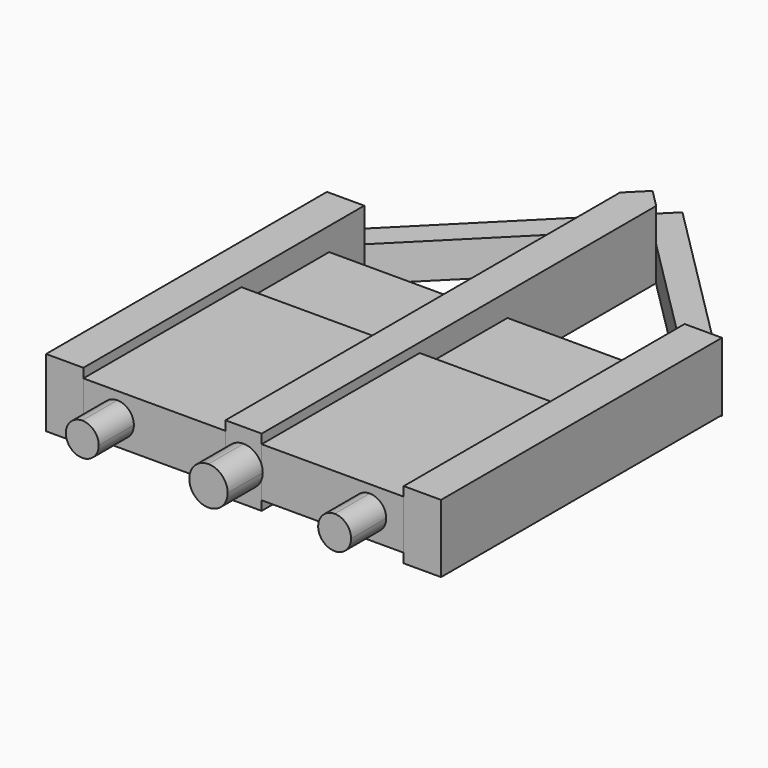
from build123d import *

# Parameters (mm, degrees)
F0_W     = 1.7
F0_H     = 9
F0_H_2   = 2
F0_H_3   = 5
F1_DEPTH = 1.55
F0_W_2   = 0.825
F2_DEPTH = 1.125
F3_DEPTH = 1.6
F0_W_3   = 6.475
F4_DEPTH = 0.5
F0_W_4   = 1.5
F5_DEPTH = 0.75
F6_DEPTH = 0.875
F7_R     = 0.87499
F8_R     = 0.74999
F8_2_R   = 0.74999


# Not quite as in the source:
# - a fillet or chamfer is up to 0.001 mm smaller than in the source, because OpenCascade refuses the exact size


with BuildPart() as f1:
    # F0 (on Top) → F1 (new body, symmetric)
    with BuildSketch(Plane.XY):
        with Locations((0.85, 4.5)):
            Rectangle(F0_W, F0_H)
        with Locations((0.85, 15)):
            Rectangle(F0_W, F0_H_2)
        with Locations((0.85, 11.5)):
            Rectangle(F0_W, F0_H_3)
    extrude(amount=F1_DEPTH, both=True)


with BuildPart() as f1b:
    # F0 (on Top) → F1, piece 2 (new body, symmetric)
    with BuildSketch(Plane.XY):
        with Locations((17.15, 4.5)):
            Rectangle(F0_W, F0_H)
        with Locations((17.15, 15)):
            Rectangle(F0_W, F0_H_2)
        with Locations((17.15, 11.5)):
            Rectangle(F0_W, F0_H_3)
    extrude(amount=F1_DEPTH, both=True)


with BuildPart() as f1c:
    # F0 (on Top) → F1, piece 3 (new body, symmetric)
    with BuildSketch(Plane.XY):
        with Locations((8.5875, 4.5)):
            Rectangle(F0_W_2, F0_H)
        with Locations((9.4125, 4.5)):
            Rectangle(F0_W_2, F0_H)
        with Locations((9.4125, 11.5)):
            Rectangle(F0_W_2, F0_H_3)
        with Locations((8.5875, 11.5)):
            Rectangle(F0_W_2, F0_H_3)
        Polygon((8.175, 22.475), (8.175, 14), (9, 14), (9, 23.3), align=None)
        Polygon((9, 23.3), (9, 14), (9.825, 14), (9.825, 22.475), align=None)
    extrude(amount=F1_DEPTH, both=True)


with BuildPart() as f2:
    # F0 (on Top) → F2 (new body, symmetric)
    with BuildSketch(Plane.XY):
        Polygon((1.7, 9), (1.7, 0), (2.5, 0), (4, 0), (8.125, 0), (8.175, 0), (8.175, 9), align=None)
    extrude(amount=F2_DEPTH, both=True)


with BuildPart() as f2b:
    # F0 (on Top) → F2, piece 2 (new body, symmetric)
    with BuildSketch(Plane.XY):
        Polygon((16.3, 9), (9.825, 9), (9.825, 0), (9.875, 0), (14, 0), (15.5, 0), (16.3, 0), align=None)
    extrude(amount=F2_DEPTH, both=True)


with BuildPart() as f3:
    # F0 (on Top) → F3 (new body)
    with BuildSketch(Plane.XY):
        Polygon((9, 25), (0, 16), (1.7, 16), (8.175, 22.475), (9, 23.3), align=None)
        Polygon((18, 16), (9, 25), (9, 23.3), (9.825, 22.475), (16.3, 16), align=None)
    extrude(amount=-F3_DEPTH)


with BuildPart() as f4:
    # F0 (on Top) → F4 (new body, symmetric)
    with BuildSketch(Plane.XY):
        with Locations((4.9375, 11.5)):
            Rectangle(F0_W_3, F0_H_3)
    extrude(amount=F4_DEPTH, both=True)


with BuildPart() as f4b:
    # F0 (on Top) → F4, piece 2 (new body, symmetric)
    with BuildSketch(Plane.XY):
        with Locations((13.0625, 11.5)):
            Rectangle(F0_W_3, F0_H_3)
    extrude(amount=F4_DEPTH, both=True)


with BuildPart() as f5:
    # F0 (on Top) → F5 (new body, symmetric)
    with BuildSketch(Plane.XY):
        with Locations((3.25, -1)):
            Rectangle(F0_W_4, F0_H_2)
    extrude(amount=F5_DEPTH, both=True)

    # F8#2 (radius 0.75 in the source; OpenCascade refuses exactly that, so slightly less here)
    f8_2_edges = [f5.edges().sort_by_distance(p)[0] for p in [
        (2.5, -1, 0.75),
        (4, -1, 0.75),
        (2.5, -1, -0.75),
        (4, -1, -0.75),
    ]]
    fillet(f8_2_edges, radius=F8_2_R)


with BuildPart() as f5b:
    # F0 (on Top) → F5, piece 2 (new body, symmetric)
    with BuildSketch(Plane.XY):
        with Locations((14.75, -1)):
            Rectangle(F0_W_4, F0_H_2)
    extrude(amount=F5_DEPTH, both=True)

    # F8 (radius 0.75 in the source; OpenCascade refuses exactly that, so slightly less here)
    f8_edges = [f5b.edges().sort_by_distance(p)[0] for p in [
        (14, -1, 0.75),
        (15.5, -1, 0.75),
        (15.5, -1, -0.75),
        (14, -1, -0.75),
    ]]
    fillet(f8_edges, radius=F8_R)


with BuildPart() as f6:
    # F0 (on Top) → F6 (new body, symmetric)
    with BuildSketch(Plane.XY):
        Polygon((8.175, 0), (8.125, 0), (8.125, -2), (9.875, -2), (9.875, 0), (9.825, 0), (9, 0), align=None)
    extrude(amount=F6_DEPTH, both=True)

    # F7 (radius 0.875 in the source; OpenCascade refuses exactly that, so slightly less here)
    f7_edges = [f6.edges().sort_by_distance(p)[0] for p in [
        (9.875, -1, -0.875),
        (8.125, -1, -0.875),
        (9.875, -1, 0.875),
        (8.125, -1, 0.875),
    ]]
    fillet(f7_edges, radius=F7_R)


solid = Compound([f1.part, f1b.part, f1c.part, f2.part, f2b.part, f3.part, f4.part, f4b.part, f5.part, f5b.part, f6.part])
